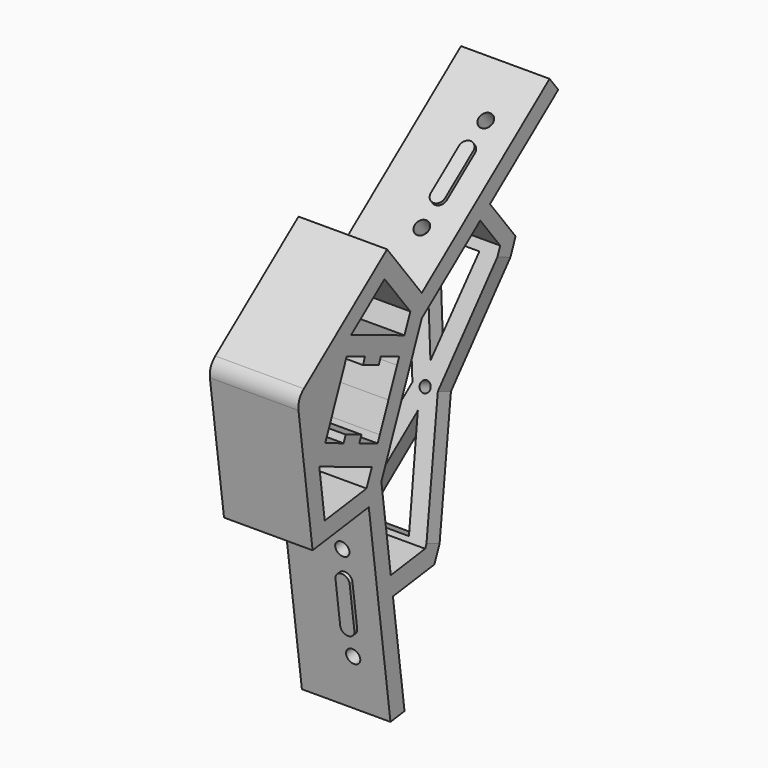
from build123d import *

# Parameters (mm, degrees)
F1_DEPTH  = 25
F2_DEPTH  = 5
F3_R      = 5
F5_DEPTH  = 5
F6_W      = 25
F6_H      = 37.5846914337
F10_R     = 1.55
F11_DEPTH = 10
F14_DEPTH = 1
F15_DEPTH = 1
F16_DEPTH = 5
F17_DEPTH = 5


# Not quite as in the source:
# - a feature names something its author has since deleted; it is built from what else it names


with BuildPart() as f1:
    # F0 (on Right) → F1 (new body)
    with BuildSketch(Plane.YZ):
        Polygon((-1.9545168432, 38.6489601963), (-33.5964987424, 14.1788767986), (-28.2257758369, -25.4589250511), (-8.406874912, -22.7735635983), (-0.7535947717, -79.2574312341), (4.2011304595, -78.5860908709), (0.1149024355, -48.4283077234), (-0.6409071668, -42.8501701471), (-3.9713255886, -18.2705245759), (3.1545996335, -0.8816359607), (10.2805248557, 16.5072526545), (30.8972257421, 32.4510197574), (34.3548171712, 35.1249215027), (58.4291094867, 53.742590351), (55.370349062, 57.6978380884), (10.2805248557, 22.8279692467), align=None)
        Polygon((-25.8654488138, -5.6400241263), (-7.3142972833, -13.2422419285), (-9.1963342424, -17.8348428934), (-23.9423909688, -19.8328594567), align=None, mode=Mode.SUBTRACT)
        Polygon((1.5615552233, 8.4168698067), (-1.4719884671, 1.0143288458), (-4.5055321574, -6.3882121151), (-5.26391808, -8.2388473554), (-11.7411414209, -5.5844966263), (-17.2930471416, -3.3093388585), (-23.7702704824, -0.6549881294), (-23.0118845598, 1.1956471108), (-16.944797179, 16.0007290327), (-16.1864112564, 17.851364273), (-9.7091879156, 15.1970135439), (-4.1572821949, 12.9218557761), (2.3199411459, 10.267505047), align=None, mode=Mode.SUBTRACT)
        Polygon((-14.6534166938, 22.50764705), (-2.8510041559, 31.6349520341), (6.2523573083, 19.863500585), (4.1741345282, 14.7921613112), align=None, mode=Mode.SUBTRACT)
        Polygon((-10.4675738382, 13.3463783036), (-4.9156681175, 11.0712205358), (-4.1572821949, 12.9218557761), (-9.7091879156, 15.1970135439), align=None)
        Polygon((-11.7411414209, -5.5844966263), (-10.9827554983, -3.7338613861), (-16.534661219, -1.4587036183), (-17.2930471416, -3.3093388585), align=None)
        Polygon((43.3848339814, 23.4483111776), (34.3548171712, 35.1249215027), (30.8972257421, 32.4510197574), (37.9390681356, 23.3452947817), (11.4856577492, -41.2070815569), (-0.6409071668, -42.8501701471), (0.1149024355, -48.4283077234), (14.7421520123, -46.4463889317), align=None)
    extrude(amount=F1_DEPTH)

    # F0 (on Right) → F2 (join)
    with BuildSketch(Plane.YZ):
        Polygon((-16.944797179, 16.0007290327), (-10.4675738382, 13.3463783036), (-9.7091879156, 15.1970135439), (-16.1864112564, 17.851364273), align=None)
        Polygon((-4.9156681175, 11.0712205358), (1.5615552233, 8.4168698067), (2.3199411459, 10.267505047), (-4.1572821949, 12.9218557761), align=None)
        Polygon((-17.2930471416, -3.3093388585), (-16.534661219, -1.4587036183), (-23.0118845598, 1.1956471108), (-23.7702704824, -0.6549881294), align=None)
        Polygon((-5.26391808, -8.2388473554), (-4.5055321574, -6.3882121151), (-10.9827554983, -3.7338613861), (-11.7411414209, -5.5844966263), align=None)
    extrude(amount=F2_DEPTH)

    # F3
    f3_edges = [f1.edges().sort_by_distance(p)[0] for p in [
        (12.5, -33.596499, 14.178877),
    ]]
    fillet(f3_edges, radius=F3_R)

    # F4 (on face) → F5 (cut)
    with BuildSketch(Plane(origin=(0, 28.9192447, -11.8510377387), x_dir=(-1, 0, 0), z_dir=(0, 0.9253176201, -0.3791929613))):
        Polygon((-25, 33.3185826418), (-25, -32.5577652662), (-18.2082508509, 0.3804086878), align=None)
        Polygon((-14.2606471901, -5.2335595779), (-20, -32.3875417919), (-4.8253758508, -32.3875417919), align=None)
        Polygon((-11.0385, 0.3804086878), (0, -31.3875417919), (0, 32.1483591675), align=None)
        with BuildLine():
            ThreePointArc((-13.1233754255, 0.3804086878), (-14.6233754255, 1.8804086878), (-16.1233754255, 0.3804086878))
            Line((-16.1233754255, 0.3804086878), (-13.1233754255, 0.3804086878))
        make_face()
        with BuildLine():
            Line((-13.1233754255, 0.3804086878), (-16.1233754255, 0.3804086878))
            ThreePointArc((-16.1233754255, 0.3804086878), (-14.6233754255, -1.1195913122), (-13.1233754255, 0.3804086878))
        make_face()
        Polygon((-5, 33.1483591675), (-20, 33.1483591675), (-14.3256804669, 6.3097710203), align=None)
    extrude(amount=-F5_DEPTH, mode=Mode.SUBTRACT)

    # F8 (on offset) → F9 section 0
    with BuildSketch(Plane(origin=(0, 12.2635275379, -5.0255644353), x_dir=(-1, 0, 0), z_dir=(0, 0.9253176201, -0.3791929613))):
        with BuildLine():
            ThreePointArc((-17.1248646707, 2.8558931882), (-18.1499909365, 0.381019454), (-17.1248646707, -2.0938542801))
            ThreePointArc((-17.1248646707, -2.0938542801), (-14.6499909365, -3.118980546), (-12.1751172024, -2.0938542801))
            ThreePointArc((-12.1751172024, -2.0938542801), (-11.1499909365, 0.381019454), (-12.1751172024, 2.8558931882))
            ThreePointArc((-12.1751172024, 2.8558931882), (-14.6499909365, 3.881019454), (-17.1248646707, 2.8558931882))
        make_face()
    # F6 (on face) → F9 section 1
    with BuildSketch(Plane(origin=(0, 3.0103513367, -1.2336348224), x_dir=(-1, 0, 0), z_dir=(0, 0.9253176201, -0.3791929613))):
        with Locations((-12.5, 0.3804086878)):
            Rectangle(F6_W, F6_H)
    loft()

    # F10 (on face) → F11 (cut)
    with BuildSketch(Plane(origin=(0, 12.2635275379, -5.0255644353), x_dir=(-1, 0, 0), z_dir=(0, 0.9253176201, -0.3791929613))):
        with Locations((-14.6499909461, 0.3810196067)):
            Circle(F10_R)
    extrude(amount=-F11_DEPTH, mode=Mode.SUBTRACT)

    # F13 (on face) → F14 (join)
    with BuildSketch(Plane(origin=(0, -11.2853910764, -1.5291137632), x_dir=(1, 0, 0), z_dir=(0, -0.9909450462, -0.1342680726))):
        with BuildLine():
            ThreePointArc((14, -43.6885751417), (16, -45.6885751417), (18, -43.6885751417))
            ThreePointArc((18, -43.6885751417), (16, -41.6885751417), (14, -43.6885751417))
        make_face()
        with BuildLine():
            Line((18, -56.1885751417), (18, -43.6885751417))
            ThreePointArc((18, -43.6885751417), (16, -45.6885751417), (14, -43.6885751417))
            Line((14, -43.6885751417), (14, -56.1885751417))
            ThreePointArc((14, -56.1885751417), (16, -54.1885751417), (18, -56.1885751417))
        make_face()
        with BuildLine():
            ThreePointArc((14, -56.1885751417), (16, -58.1885751417), (18, -56.1885751417))
            ThreePointArc((18, -56.1885751417), (16, -54.1885751417), (14, -56.1885751417))
        make_face()
    extrude(amount=F14_DEPTH)

    # F12 (on face) → F15 (join)
    with BuildSketch(Plane(origin=(0, -7.1996627103, 9.3098006026), x_dir=(1, 0, 0), z_dir=(0, -0.6117520849, 0.7910495475))):
        with BuildLine():
            ThreePointArc((14, 56.8474623166), (16, 54.8474623166), (18, 56.8474623166))
            ThreePointArc((18, 56.8474623166), (16, 58.8474623166), (14, 56.8474623166))
        make_face()
        with BuildLine():
            Line((18, 44.3474623166), (18, 56.8474623166))
            ThreePointArc((18, 56.8474623166), (16, 54.8474623166), (14, 56.8474623166))
            Line((14, 56.8474623166), (14, 44.3474623166))
            ThreePointArc((14, 44.3474623166), (16, 46.3474623166), (18, 44.3474623166))
        make_face()
        with BuildLine():
            ThreePointArc((14, 44.3474623166), (16, 42.3474623166), (18, 44.3474623166))
            ThreePointArc((18, 44.3474623166), (16, 46.3474623166), (14, 44.3474623166))
        make_face()
    extrude(amount=F15_DEPTH)

    # F12 (on face) → F16 (cut)
    with BuildSketch(Plane(origin=(0, -7.1996627103, 9.3098006026), x_dir=(1, 0, 0), z_dir=(0, -0.6117520849, 0.7910495475))):
        with BuildLine():
            ThreePointArc((14, 64.8474623166), (16, 62.8474623166), (18, 64.8474623166))
            ThreePointArc((18, 64.8474623166), (16, 66.8474623166), (14, 64.8474623166))
        make_face()
        with BuildLine():
            ThreePointArc((14, 36.3474623166), (16, 34.3474623166), (18, 36.3474623166))
            ThreePointArc((18, 36.3474623166), (16, 38.3474623166), (14, 36.3474623166))
        make_face()
    extrude(amount=-F16_DEPTH, mode=Mode.SUBTRACT)

    # F13 (on face) → F17 (cut)
    with BuildSketch(Plane(origin=(0, -11.2853910764, -1.5291137632), x_dir=(1, 0, 0), z_dir=(0, -0.9909450462, -0.1342680726))):
        with BuildLine():
            ThreePointArc((14, -35.6885751417), (16, -37.6885751417), (18, -35.6885751417))
            ThreePointArc((18, -35.6885751417), (16, -33.6885751417), (14, -35.6885751417))
        make_face()
        with BuildLine():
            ThreePointArc((14, -64.1885751417), (16, -66.1885751417), (18, -64.1885751417))
            ThreePointArc((18, -64.1885751417), (16, -62.1885751417), (14, -64.1885751417))
        make_face()
    extrude(amount=-F17_DEPTH, mode=Mode.SUBTRACT)


solid = f1.part
